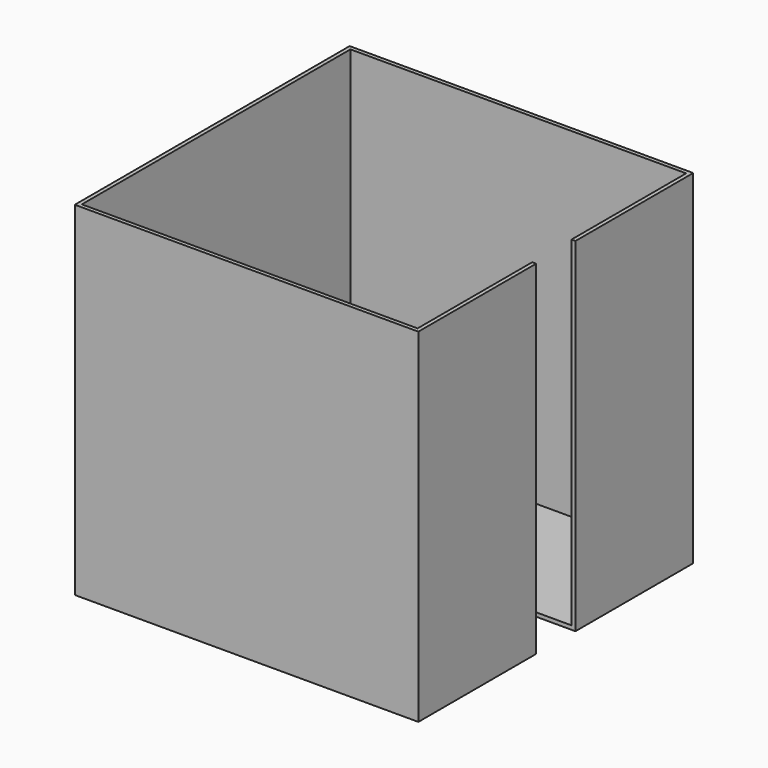
from build123d import *

# Parameters (mm, degrees)
F1_DEPTH = 44.45
F2_T     = -0.508


# Not quite as in the source:
# - the program builds the solid bodies; features that only make, move or delete a surface that nothing else refers to are left out


with BuildPart() as f1:
    # F0 (on Top) → F1 (new body)
    with BuildSketch(Plane.XY):
        Polygon((0, 44.45), (0, 0), (44.45, 0), (44.45, 19.05), (22.225, 19.05), (22.225, 25.4), (44.45, 25.4), (44.45, 44.45), align=None)
    extrude(amount=F1_DEPTH)

    # F2
    f2_openings = [f1.faces().sort_by_distance(p)[0] for p in [
        (21.370192, 22.225, 44.45),
        (22.225, 22.225, 22.225),
        (33.3375, 25.4, 22.225),
        (33.3375, 19.05, 22.225),
    ]]
    offset(amount=F2_T, openings=f2_openings)


solid = f1.part
